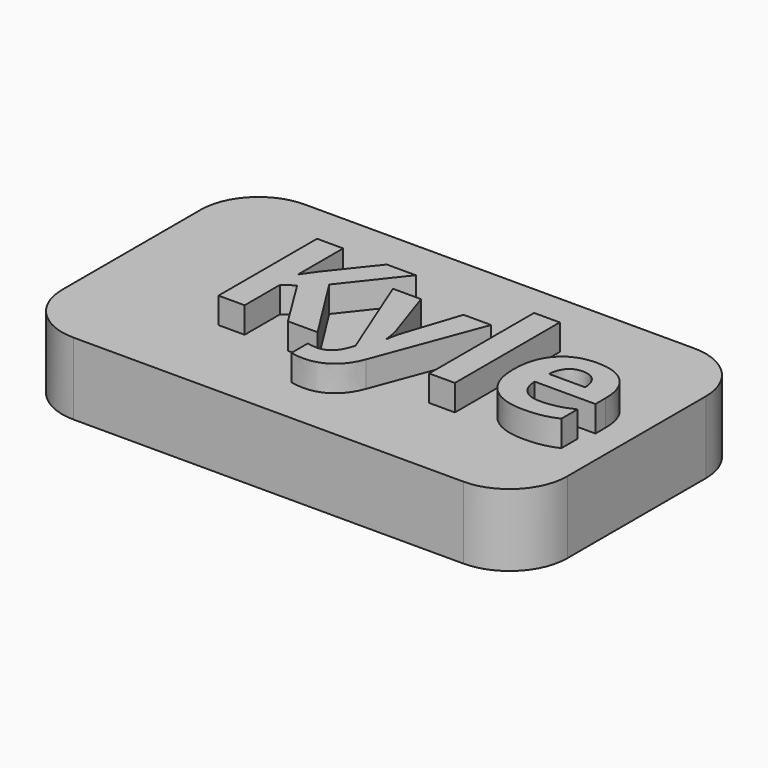
from build123d import *

# Parameters (mm, degrees)
F0_W         = 44.45
F0_H         = 25.4
F1_DEPTH     = 6.35
F2_TEXT_SIZE = 15.1827776184
F3_DEPTH     = 2.286
F6_R         = 5.08


# Not quite as in the source:
# - the program builds the solid bodies; features that only make, move or delete a surface that nothing else refers to are left out
# - Text() gives the source's letters only with a copy of the font that has no kerning and outlines rounded to 1/6400 em; it was checked with that copy


with BuildPart() as f1:
    # F0 (on Top) → F1 (new body)
    with BuildSketch(Plane.XY):
        with Locations((-40.8892035842, 39.6801169634)):
            Rectangle(F0_W, F0_H)
    extrude(amount=F1_DEPTH)

    # F2 (on face) → F3 (join)
    with BuildSketch(Plane.XY.offset(6.35)):
        with Locations((-52.7972988784, 34.6554927528)):
            Text('Kyle', F2_TEXT_SIZE, font='Open Sans', font_style=FontStyle.BOLD, text_align=(TextAlign.LEFT, TextAlign.BOTTOM))
    extrude(amount=F3_DEPTH)

    # F6
    f6_edges = [f1.edges().sort_by_distance(p)[0] for p in [
        (-63.114204, 52.380117, 3.175),
        (-18.664204, 52.380117, 3.175),
        (-18.664204, 26.980117, 3.175),
        (-63.114204, 26.980117, 3.175),
    ]]
    fillet(f6_edges, radius=F6_R)


solid = f1.part
